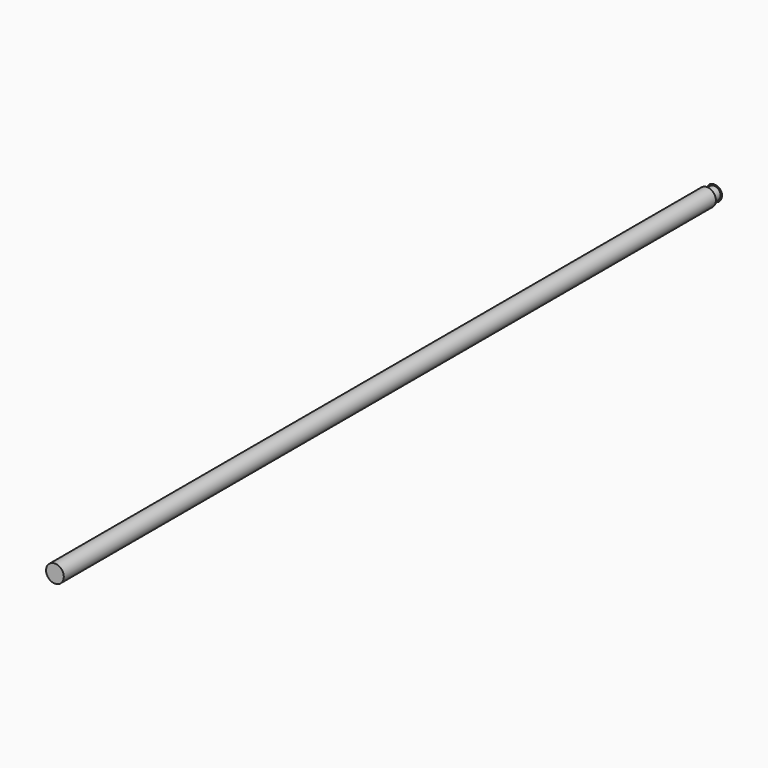
from build123d import *

# Parameters (mm, degrees)
F0_R     = 6.35
F1_DEPTH = 584.2
F2_R     = 4.6163674118
F3_DEPTH = 6.35
F4_R     = 5.5303676916
F5_DEPTH = 2.54


# Not quite as in the source:
# - a fillet or chamfer that OpenCascade refuses, or shapes differently, is made with other operations: its cross-section is extruded or revolved along the edge and cut away or added


with BuildPart() as f1:
    # F0 (on Front) → F1 (new body)
    with BuildSketch(Plane.XZ):
        Circle(F0_R)
    extrude(amount=F1_DEPTH)


with BuildPart() as f3:
    # F2 (on face) → F3 (new body)
    with BuildSketch(Plane(origin=(0, 0, 0), x_dir=(-1, 0, 0), z_dir=(0, 1, 0))):
        Circle(F2_R)
    extrude(amount=F3_DEPTH)

    # F4 (on face) → F5 (join)
    with BuildSketch(Plane(origin=(0, 6.35, 0), x_dir=(-1, 0, 0), z_dir=(0, 1, 0))):
        Circle(F4_R)
    extrude(amount=F5_DEPTH)

    # F6: fillet of radius 5.08 on 1 edges, made by hand

    # F6_s1 → F6_t2 (revolve, cut)
    with BuildSketch(Plane.XY):
        with BuildLine():
            ThreePointArc((-5.5303676916, 6.35), (-3.6709586404, 8.2094090512), (-1.1309586404, 8.89))
            Line((-1.1309586404, 8.89), (-5.5303676916, 8.89))
            Line((-5.5303676916, 8.89), (-5.5303676916, 6.35))
        make_face()
    revolve(axis=Axis((0, 8.89, 0), (0, 1, 0)), mode=Mode.SUBTRACT)


solid = Compound([f1.part, f3.part])
